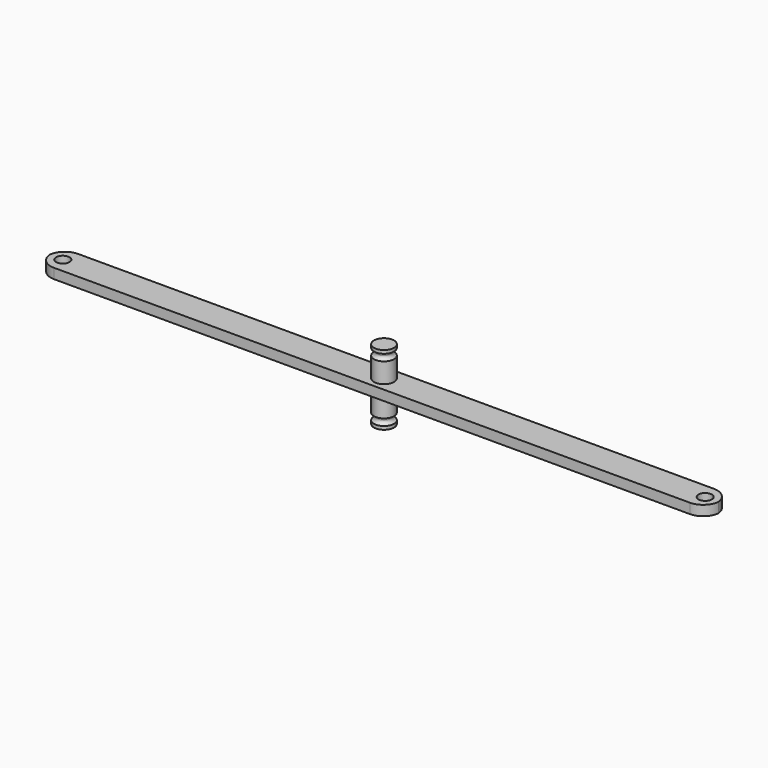
from build123d import *

# Parameters (mm, degrees)
F0_W        = 200
F0_H        = 9
F1_DEPTH    = 3
F2_R        = 2
F3_DEPTH    = 25
F4_T1_DEPTH = 28
F5_R        = 3
F6_DEPTH    = 9
F8_R        = 1


# Not quite as in the source:
# - a fillet or chamfer that OpenCascade refuses, or shapes differently, is made with other operations: its cross-section is extruded or revolved along the edge and cut away or added


with BuildPart() as f1:
    # F0 (on Top) → F1 (new body)
    with BuildSketch(Plane.XY):
        Rectangle(F0_W, F0_H)
    extrude(amount=F1_DEPTH)

    # F2 (on face) → F3 (cut)
    with BuildSketch(Plane(origin=(0, 0, 0), x_dir=(1, 0, 0), z_dir=(0, 0, -1))):
        with Locations((-96, 0)):
            Circle(F2_R)
        with Locations((96, 0)):
            Circle(F2_R)
    extrude(amount=-F3_DEPTH, mode=Mode.SUBTRACT)

    # F4: fillet of radius 5 on 4 edges, made by hand

    # F4_s2 → F4_t1 (cut)
    with BuildSketch(Plane.XY.offset(-12.5)):
        with BuildLine():
            ThreePointArc((95, 4.5), (98.5355339059, 3.0355339059), (100, -0.5))
            Line((100, -0.5), (100, 4.5))
            Line((100, 4.5), (95, 4.5))
        make_face()
        with BuildLine():
            ThreePointArc((100, 0.5), (98.5355339059, -3.0355339059), (95, -4.5))
            Line((95, -4.5), (100, -4.5))
            Line((100, -4.5), (100, 0.5))
        make_face()
        with BuildLine():
            ThreePointArc((-95, 4.5), (-98.5355339059, 3.0355339059), (-100, -0.5))
            Line((-100, -0.5), (-100, 4.5))
            Line((-100, 4.5), (-95, 4.5))
        make_face()
        with BuildLine():
            ThreePointArc((-100, 0.5), (-98.5355339059, -3.0355339059), (-95, -4.5))
            Line((-95, -4.5), (-100, -4.5))
            Line((-100, -4.5), (-100, 0.5))
        make_face()
    extrude(amount=F4_T1_DEPTH, mode=Mode.SUBTRACT)

    # F5 (on face) → F6 (join)
    with BuildSketch(Plane.XY.offset(3)):
        Circle(F5_R)
    extrude(amount=F6_DEPTH)

    # F8 (on face) → F9 (revolve, cut)
    with BuildSketch(Plane(origin=(0, 0, 0), x_dir=(-1, 0, 0), z_dir=(0, 1, 0))):
        with Locations((-3, 10)):
            Circle(F8_R)
    revolve(axis=Axis((0, 0, 12), (0, 0, 1)), mode=Mode.SUBTRACT)

    # F14: F1 across plane


with BuildPart() as f1_1:
    add(f1.part)
    add(f1.part.mirror(Plane(origin=(95, -4.5, 1.5), x_dir=(-1, 0, 0), z_dir=(0, 0, 1))))


solid = f1_1.part
